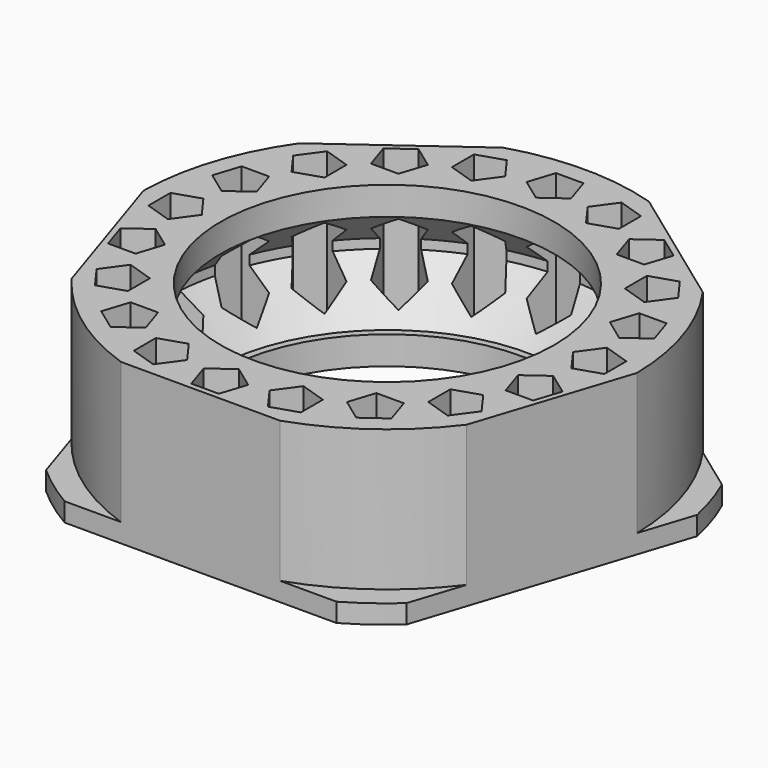
from build123d import *

# Parameters (mm, degrees)
F0_R            = 26.25
F0_R_2          = 17.75
F1_DEPTH        = 17
F0_R_3          = 28.75
F2_DEPTH        = 2
F4_R            = 23.5194172772
F5_DEPTH        = 5.5
F6_SIZE         = 5
F8_DEPTH        = 20
F8_COPIES_COUNT = 20
F9_DEPTH        = 29.9
F9_COPIES_COUNT = 5


# Not quite as in the source:
# - a pattern or mirror of a feature is missing from the dataset's text; its kind, count and spacing are read off the source's solid


with BuildPart() as f1:
    # F0 (on Top) → F1 (new body)
    with BuildSketch(Plane.XY):
        Circle(F0_R)
        Circle(F0_R_2, mode=Mode.SUBTRACT)
    extrude(amount=F1_DEPTH)

    # F0 (on Top) → F2 (join)
    with BuildSketch(Plane.XY):
        Circle(F0_R_3)
        Circle(F0_R, mode=Mode.SUBTRACT)
    extrude(amount=F2_DEPTH)

    # F4 (on offset) → F5 (cut, symmetric)
    with BuildSketch(Plane.XY.offset(8.5)):
        Circle(F4_R)
    extrude(amount=F5_DEPTH, both=True, mode=Mode.SUBTRACT)

    # F6
    f6_edges = [f1.edges().sort_by_distance(p)[0] for p in [
        (-23.519417, 0, 3),
        (-23.519417, 0, 14),
    ]]
    chamfer(f6_edges, length=F6_SIZE)

    # F7 (on face) → F8 (cut)
    with BuildSketch(Plane.XY.offset(17)):
        Polygon((1.462138633, 24.25), (-1.462138633, 24.25), (-2.3657900045, 21.4688470506), (0, 19.75), (2.3657900045, 21.4688470506), align=None)
    f8 = extrude(amount=-F8_DEPTH, mode=Mode.SUBTRACT)

    # F8_copies: F8 ×20 about axis
    f8_copies_axis = Axis((0, 0, 0), (0, 0, 1))
    for i in range(1, F8_COPIES_COUNT):
        add(f8.rotate(f8_copies_axis, i * 360 / F8_COPIES_COUNT), mode=Mode.SUBTRACT)

    # F7 (on face) → F9 (cut)
    with BuildSketch(Plane.XY.offset(17)):
        with BuildLine():
            Line((-8.4581321815, -24.85), (-28.9675127715, -24.85))
            Line((-28.9675127715, -24.85), (-28.9675127715, -43.5834790826))
            Line((-28.9675127715, -43.5834790826), (28.9675127715, -43.5834790826))
            Line((28.9675127715, -43.5834790826), (28.9675127715, -24.85))
            Line((28.9675127715, -24.85), (8.4581321815, -24.85))
            ThreePointArc((8.4581321815, -24.85), (0, -26.25), (-8.4581321815, -24.85))
        make_face()
        with BuildLine():
            Line((8.4581321815, -24.85), (-8.4581321815, -24.85))
            ThreePointArc((-8.4581321815, -24.85), (0, -26.25), (8.4581321815, -24.85))
        make_face()
    f9 = extrude(amount=-F9_DEPTH, mode=Mode.SUBTRACT)

    # F9_copies: F9 ×5 about axis
    f9_copies_axis = Axis((0, 0, 0), (0, 0, 1))
    for i in range(1, F9_COPIES_COUNT):
        add(f9.rotate(f9_copies_axis, i * 360 / F9_COPIES_COUNT), mode=Mode.SUBTRACT)


solid = f1.part
